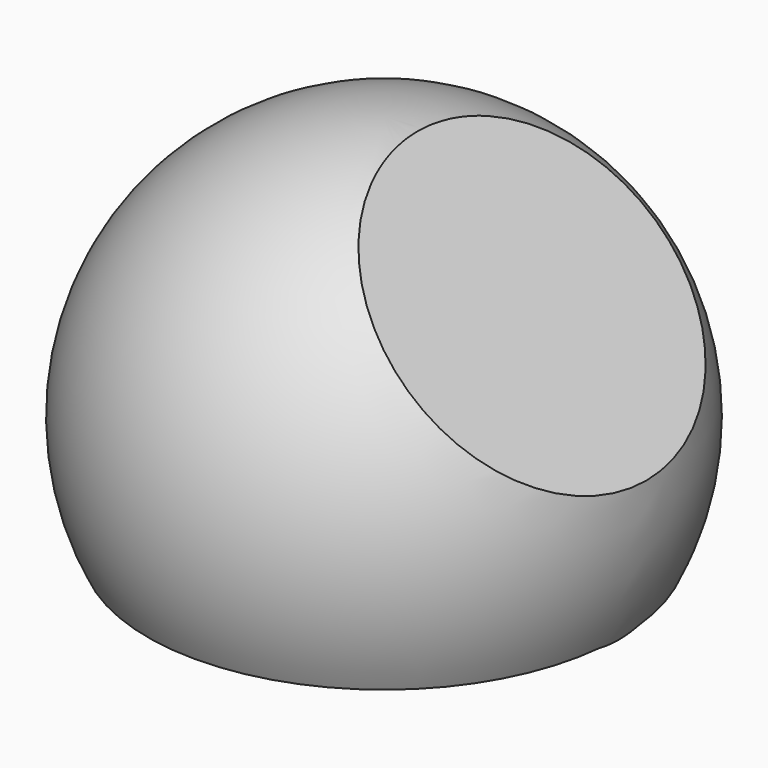
from build123d import *

# Parameters (mm, degrees)
F4_DEPTH      = 45.391737605
F4_DEPTH_BACK = 45.391737605
F6_DEPTH      = 45.391737605
F7_DEPTH      = 45.391737605


with BuildPart() as f2:
    # F0 (on Front) → F2 (revolve)
    with BuildSketch(Plane.XZ):
        with BuildLine():
            Line((0, 45.390737605), (0, -45.390737605))
            ThreePointArc((0, -45.390737605), (45.390737605, 0), (0, 45.390737605))
        make_face()
    revolve(axis=Axis((0, 0, -0.1771636307), (0, 0, -1)))

    # F3 (on Front) → F4 (cut, two sides)
    with BuildSketch(Plane.XZ) as f4_sk:
        Polygon((0, -20.2791038901), (-40.3937026858, -20.2791038901), (-40.3937026858, -45.9680799395), (0, -45.9680799395), (40.3937026858, -45.9680799395), (40.3937026858, -20.2791038901), align=None)
    extrude(amount=-F4_DEPTH, mode=Mode.SUBTRACT)
    extrude(f4_sk.sketch, amount=F4_DEPTH_BACK, mode=Mode.SUBTRACT)

    # F5 (on Front) → F6 (cut, through all)
    with BuildSketch(Plane.XZ):
        Polygon((9.3581555411, 46.5339459479), (4.3016839772, 46.5339459479), (47.9137524962, 2.0791364368), (50.4419840872, 46.5339459479), align=None)
    extrude(amount=F6_DEPTH, mode=Mode.SUBTRACT)

    # F5 (on Front) → F7 (cut, through all)
    with BuildSketch(Plane.XZ):
        Polygon((9.3581555411, 46.5339459479), (4.3016839772, 46.5339459479), (47.9137524962, 2.0791364368), (50.4419840872, 46.5339459479), align=None)
    extrude(amount=-F7_DEPTH, mode=Mode.SUBTRACT)


solid = f2.part
